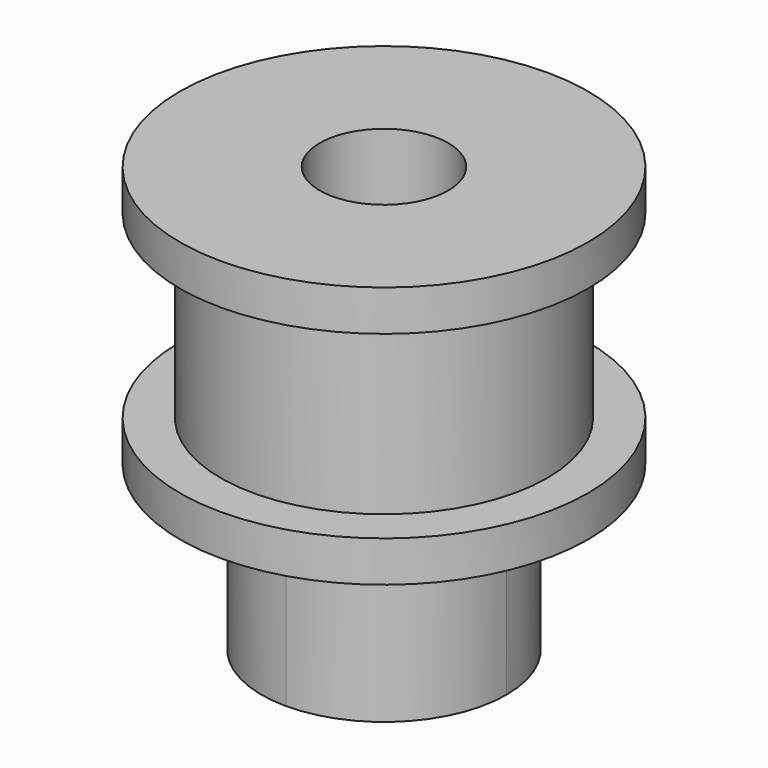
from build123d import *

# Parameters (mm, degrees)
F0_R         = 6.35
F1_DEPTH     = 7
F2_R         = 7.9375
F3_DEPTH     = 1.5875
F4_R         = 7.9375
F5_DEPTH     = 1.5875
F6_W         = 9.525
F6_H         = 9.525
F7_DEPTH     = 6.35
F8_R         = 2.5
F9_DEPTH     = 16.525
F11_REACH    = 16.5631366107
F12_T1_DEPTH = 18.25625


# Not quite as in the source:
# - a fillet or chamfer that OpenCascade refuses, or shapes differently, is made with other operations: its cross-section is extruded or revolved along the edge and cut away or added


with BuildPart() as f1:
    # F0 (on Top) → F1 (new body)
    with BuildSketch(Plane.XY):
        Circle(F0_R)
    extrude(amount=F1_DEPTH)

    # F2 (on face) → F3 (join)
    with BuildSketch(Plane.XY.offset(7)):
        Circle(F2_R)
    extrude(amount=F3_DEPTH)

    # F4 (on face) → F5 (join)
    with BuildSketch(Plane(origin=(0, 0, 0), x_dir=(1, 0, 0), z_dir=(0, 0, -1))):
        Circle(F4_R)
    extrude(amount=F5_DEPTH)

    # F6 (on face) → F7 (join)
    with BuildSketch(Plane(origin=(0, 0, -1.5875), x_dir=(1, 0, 0), z_dir=(0, 0, -1))):
        Rectangle(F6_W, F6_H)
    extrude(amount=F7_DEPTH)

    # F8 (on face) → F9 (cut, through all)
    with BuildSketch(Plane(origin=(0, 0, -7.9375), x_dir=(1, 0, 0), z_dir=(0, 0, -1))):
        Circle(F8_R)
    extrude(amount=-F9_DEPTH, mode=Mode.SUBTRACT)

    f11_end = f1.faces().sort_by_distance((-2.5, 0, 0.325))[0]
    # F10 (on face) → F11 (cut, up to a face of the model that its end follows)
    with BuildSketch(Plane(origin=(-4.7625, 0, 0), x_dir=(0, -1, 0), z_dir=(-1, 0, 0))):
        with BuildLine():
            ThreePointArc((0, -3.0353), (-1.7272, -4.7625), (0, -6.4897))
            Line((0, -6.4897), (0, -3.0353))
        make_face()
        with BuildLine():
            Line((0, -3.0353), (0, -6.4897))
            ThreePointArc((0, -6.4897), (1.2213148325, -5.9838148325), (1.7272, -4.7625))
            ThreePointArc((1.7272, -4.7625), (1.2213148325, -3.5411851675), (0, -3.0353))
        make_face()
    f11_long = extrude(amount=-F11_REACH, mode=Mode.PRIVATE)
    add(split(f11_long, bisect_by=f11_end, keep=Keep.ALL, mode=Mode.PRIVATE).solids().sort_by_distance((-4.7625, 0, -4.7625))[0], mode=Mode.SUBTRACT)

    # F12: fillet of radius 4.7625 on 4 edges, made by hand

    # F12_s2 → F12_t1 (cut)
    with BuildSketch(Plane.XY.offset(-19.84375)):
        with BuildLine():
            ThreePointArc((-4.7625, 0), (-3.3675960454, -3.3675960454), (0, -4.7625))
            Line((0, -4.7625), (-4.7625, -4.7625))
            Line((-4.7625, -4.7625), (-4.7625, 0))
        make_face()
        with BuildLine():
            ThreePointArc((-4.7625, 0), (-3.3675960454, 3.3675960454), (0, 4.7625))
            Line((0, 4.7625), (-4.7625, 4.7625))
            Line((-4.7625, 4.7625), (-4.7625, 0))
        make_face()
        with BuildLine():
            ThreePointArc((0, 4.7625), (3.3675960454, 3.3675960454), (4.7625, 0))
            Line((4.7625, 0), (4.7625, 4.7625))
            Line((4.7625, 4.7625), (0, 4.7625))
        make_face()
        with BuildLine():
            ThreePointArc((4.7625, 0), (3.3675960454, -3.3675960454), (0, -4.7625))
            Line((0, -4.7625), (4.7625, -4.7625))
            Line((4.7625, -4.7625), (4.7625, 0))
        make_face()
    extrude(amount=F12_T1_DEPTH, mode=Mode.SUBTRACT)


solid = f1.part
